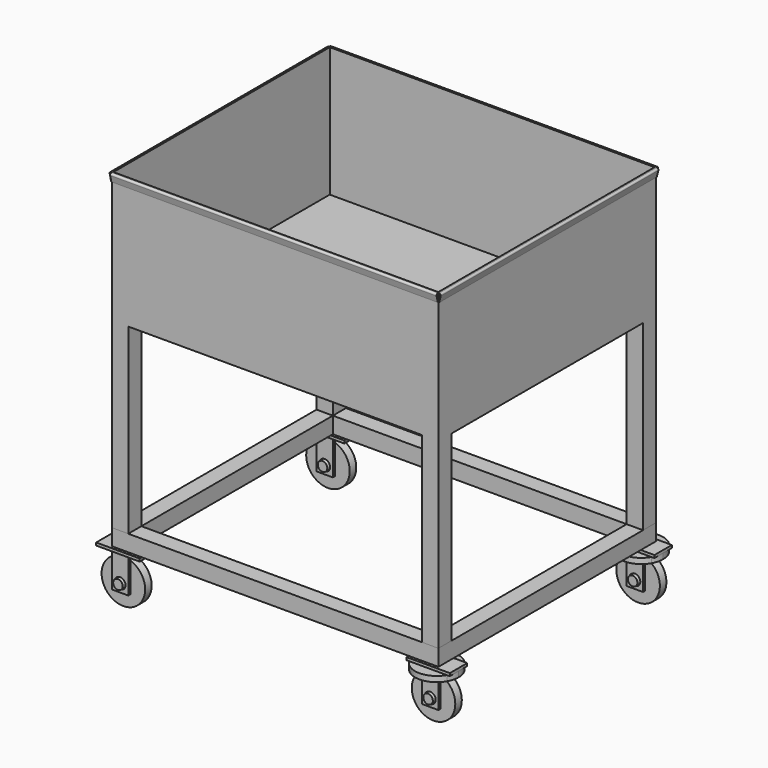
from build123d import *

# Parameters (mm, degrees)
F0_W             = 762
F0_H             = 635
F1_DEPTH         = 304.8
F2_T             = -1.89738
F3_W             = 38.1
F3_H             = 38.1
F3_W_2           = 25.4
F3_H_2           = 25.4
F4_DEPTH         = 463.8548
F5_W             = 101.6
F5_H             = 50.8
F5_W_2           = 38.1
F5_H_2           = 38.1
F5_W_3           = 25.4
F5_H_3           = 25.4
F6_DEPTH         = 6.35
F7_W             = 38.1
F7_H             = 88.9
F7_R             = 12.7
F8_DEPTH         = 6.35
F8_COPIES1_COUNT = 2
F8_COPIES1_PITCH = 724.595937
F11_R            = 50.8
F11_R_2          = 12.7
F12_DEPTH        = 9.525
F13_R            = 11.1125
F14_DEPTH        = 25.4
F18_DEPTH        = 12.7
F21_DEPTH        = 762
F23_DEPTH        = 635
F24_W            = 38.1
F24_H            = 38.1
F24_W_2          = 31.75
F24_H_2          = 6.35
F24_H_3          = 552.45
F25_DEPTH        = 38.1


# Not quite as in the source:
# - ends of sketch curves that miss each other by under 0.0002 mm in the source are joined
# - a pattern or mirror of a feature is missing from the dataset's text; its kind, count and spacing are read off the source's solid


with BuildPart() as f1:
    # F0 (on Top) → F1 (new body)
    with BuildSketch(Plane.XY):
        Rectangle(F0_W, F0_H)
    extrude(amount=F1_DEPTH)

    # F2
    f2_openings = [f1.faces().sort_by_distance(p)[0] for p in [
        (0, 0, 304.8),
    ]]
    offset(amount=F2_T, openings=f2_openings)

    # F4_copies: F4 across plane


with BuildPart() as f4:
    # F3 (on face) → F4 (new body)
    with BuildSketch(Plane(origin=(0, 0, 0), x_dir=(1, 0, 0), z_dir=(0, 0, -1))):
        with Locations((-361.95, 298.45)):
            Rectangle(F3_W, F3_H)
        with Locations((-361.95, 298.45)):
            Rectangle(F3_W_2, F3_H_2, mode=Mode.SUBTRACT)
    extrude(amount=F4_DEPTH)


with BuildPart() as f1_1:
    add(f1.part)
    add(f4.part.mirror(Plane(origin=(0, 0, 0), x_dir=(0, 0, 1), z_dir=(1, 0, 0))))

    # F6_copies: F6 across plane


with BuildPart() as f6:
    # F5 (on face) → F6 (new body)
    with BuildSketch(Plane(origin=(0, 0, -463.8548), x_dir=(1, 0, 0), z_dir=(0, 0, -1))):
        with Locations((-361.95, 298.45)):
            Rectangle(F5_W, F5_H)
        with Locations((-361.95, 298.45)):
            Rectangle(F5_W_2, F5_H_2, mode=Mode.SUBTRACT)
        with Locations((-361.95, 298.45)):
            Rectangle(F5_W_2, F5_H_2)
        with Locations((-361.95, 298.45)):
            Rectangle(F5_W_3, F5_H_3, mode=Mode.SUBTRACT)
        with Locations((-361.95, 298.45)):
            Rectangle(F5_W_3, F5_H_3)
    extrude(amount=F6_DEPTH)


with BuildPart() as f1_2:
    add(f1_1.part)
    add(f6.part.mirror(Plane(origin=(0, 0, 0), x_dir=(0, 0, 1), z_dir=(1, 0, 0))))

    # F8_copies: F8 across plane


with BuildPart() as f8:
    # F7 (on face) → F8 (new body)
    with BuildSketch(Plane.XZ.offset(317.5)):
        with Locations((-361.95, -508.3048)):
            Rectangle(F7_W, F7_H)
        with Locations((-361.95, -533.7048)):
            Circle(F7_R, mode=Mode.SUBTRACT)
    extrude(amount=-F8_DEPTH)


with BuildPart() as f1_3:
    add(f1_2.part)
    add(f8.part.mirror(Plane(origin=(0, 0, 0), x_dir=(0, 0, 1), z_dir=(1, 0, 0))))

    # F8_copies1: F8 ×2
    with Locations(*[Vector(0.9990395511, 0.0438175242, 0) * (i * F8_COPIES1_PITCH) for i in range(1, F8_COPIES1_COUNT)]):
        add(f8.part)

    # F15: F12, F8, F4, F14 across plane


with BuildPart() as f4_1:
    add(f4.part)

    add(f6.part)  # F10 merges F6
    # F10: F8 across plane
    add(f8.part.mirror(Plane(origin=(-361.95, -298.45, -467.0298), x_dir=(-1, 0, 0), z_dir=(0, 1, 0))))


with BuildPart() as f12:
    # F11 (on mid) → F12 (new body, symmetric)
    with BuildSketch(Plane(origin=(0, -298.45, 0), x_dir=(-1, 0, 0), z_dir=(0, 1, 0))):
        with Locations((361.95, -533.7048)):
            Circle(F11_R)
        with Locations((361.95, -533.7048)):
            Circle(F11_R_2, mode=Mode.SUBTRACT)
    extrude(amount=F12_DEPTH, both=True)


with BuildPart() as f14:
    # F13 (on mid) → F14 (new body, symmetric)
    with BuildSketch(Plane(origin=(0, -298.45, 0), x_dir=(-1, 0, 0), z_dir=(0, 1, 0))):
        with Locations((361.95, -533.7048)):
            Circle(F13_R)
    extrude(amount=F14_DEPTH, both=True)


with BuildPart() as f1_4:
    add(f1_3.part)
    add(f12.part.mirror(Plane.XZ))
    add(f8.part.mirror(Plane.XZ))
    add(f4_1.part.mirror(Plane.XZ))
    add(f14.part.mirror(Plane.XZ))



with BuildPart() as f1_5:
    add(f1_4.part)

    add(f4_1.part)  # F16 merges F4

    add(f8.part)  # F16 merges F8
    # F16: F12, F1, F14 across plane
    add(f12.part.mirror(Plane.YZ))
    add(f1_4.part.mirror(Plane.YZ))
    add(f14.part.mirror(Plane.YZ))


with BuildPart() as f18:
    # F17 (on face) → F18 (new body)
    with BuildSketch(Plane(origin=(0, 0, -470.2048), x_dir=(1, 0, 0), z_dir=(0, 0, -1))):
        with BuildLine():
            ThreePointArc((405.9440905122, -323.85), (411.0190319755, -311.5980074912), (412.75, -298.45))
            ThreePointArc((412.75, -298.45), (411.0190319755, -285.3019925088), (405.9440905122, -273.05))
            Line((405.9440905122, -273.05), (361.95, -273.05))
            Line((361.95, -273.05), (361.95, -279.4))
            Line((361.95, -279.4), (381, -279.4))
            Line((381, -279.4), (381, -285.75))
            Line((381, -285.75), (361.95, -285.75))
            Line((361.95, -285.75), (361.95, -311.15))
            Line((361.95, -311.15), (381, -311.15))
            Line((381, -311.15), (381, -317.5))
            Line((381, -317.5), (361.95, -317.5))
            Line((361.95, -317.5), (361.95, -323.85))
            Line((361.95, -323.85), (405.9440905122, -323.85))
        make_face()
        with BuildLine():
            Line((361.95, -273.05), (405.9440905122, -273.05))
            ThreePointArc((405.9440905122, -273.05), (361.95, -247.65), (317.9559094878, -273.05))
            Line((317.9559094878, -273.05), (361.95, -273.05))
        make_face()
        with BuildLine():
            ThreePointArc((317.9559094878, -323.85), (361.95, -349.25), (405.9440905122, -323.85))
            Line((405.9440905122, -323.85), (361.95, -323.85))
            Line((361.95, -323.85), (317.9559094878, -323.85))
        make_face()
        with BuildLine():
            Line((361.95, -273.05), (317.9559094878, -273.05))
            ThreePointArc((317.9559094878, -273.05), (312.8809680245, -285.3019925088), (311.15, -298.45))
            ThreePointArc((311.15, -298.45), (312.8809680245, -311.5980074912), (317.9559094878, -323.85))
            Line((317.9559094878, -323.85), (361.95, -323.85))
            Line((361.95, -323.85), (361.95, -317.5))
            Line((361.95, -317.5), (342.9, -317.5))
            Line((342.9, -317.5), (342.9, -311.15))
            Line((342.9, -311.15), (361.95, -311.15))
            Line((361.95, -311.15), (361.95, -285.75))
            Line((361.95, -285.75), (342.9, -285.75))
            Line((342.9, -285.75), (342.9, -279.4))
            Line((342.9, -279.4), (361.95, -279.4))
            Line((361.95, -279.4), (361.95, -273.05))
        make_face()
    extrude(amount=F18_DEPTH)


with BuildPart() as f19_1:
    # F19: instance of F18
    add(f18.part.mirror(Plane.XZ))


with BuildPart() as f21:
    # F20 (on face) → F21 (new body, through all)
    with BuildSketch(Plane(origin=(-381, 0, 0), x_dir=(0, -1, 0), z_dir=(-1, 0, 0))):
        with BuildLine():
            Line((-317.5, 302.90262), (-317.5, 304.8))
            Line((-317.5, 304.8), (-319.0535416211, 304.8))
            ThreePointArc((-319.0535416211, 304.8), (-322.0295428289, 303.359729386), (-322.7465094275, 300.1322037816))
            Line((-322.7465094275, 300.1322037816), (-319.3464839032, 285.75))
            Line((-319.3464839032, 285.75), (-317.5, 286.1865181092))
            Line((-317.5, 286.1865181092), (-320.9000255243, 300.5687218908))
            ThreePointArc((-320.9000255243, 300.5687218908), (-320.541542225, 302.182484693), (-319.0535416211, 302.90262))
            Line((-319.0535416211, 302.90262), (-317.5, 302.90262))
        make_face()
    extrude(amount=-F21_DEPTH)


with BuildPart() as f21b:
    # F20 (on face) → F21, piece 2 (new body, through all)
    with BuildSketch(Plane(origin=(-381, 0, 0), x_dir=(0, -1, 0), z_dir=(-1, 0, 0))):
        with BuildLine():
            Line((319.0535416211, 304.8), (317.5, 304.8))
            Line((317.5, 304.8), (317.5, 302.90262))
            Line((317.5, 302.90262), (319.0535416211, 302.90262))
            ThreePointArc((319.0535416211, 302.90262), (320.541542225, 302.182484693), (320.9000255243, 300.5687218908))
            Line((320.9000255243, 300.5687218908), (317.5, 286.1865181092))
            Line((317.5, 286.1865181092), (319.3464839032, 285.75))
            Line((319.3464839032, 285.75), (322.7465094275, 300.1322037816))
            ThreePointArc((322.7465094275, 300.1322037816), (322.0295428289, 303.359729386), (319.0535416211, 304.8))
        make_face()
    extrude(amount=-F21_DEPTH)


with BuildPart() as f23:
    # F22 (on face) → F23 (new body, through all)
    with BuildSketch(Plane(origin=(0, 317.5, 0), x_dir=(-1, 0, 0), z_dir=(0, 1, 0))):
        with BuildLine():
            Line((-381, 302.8843261488), (-381, 304.8))
            Line((-381, 304.8), (-383.1514110451, 304.5005266943))
            ThreePointArc((-383.1514110451, 304.5005266943), (-385.7621614566, 302.8817897377), (-386.3192742384, 299.860870607))
            Line((-386.3192742384, 299.860870607), (-382.8455219884, 285.3094328034))
            Line((-382.8455219884, 285.3094328034), (-381, 285.75))
            Line((-381, 285.75), (-384.47375225, 300.3014378036))
            ThreePointArc((-384.47375225, 300.3014378036), (-384.1951958591, 301.8118973689), (-382.8898206534, 302.6212658473))
            Line((-382.8898206534, 302.6212658473), (-381, 302.8843261488))
        make_face()
    extrude(amount=-F23_DEPTH)


with BuildPart() as f23b:
    # F22 (on face) → F23, piece 2 (new body, through all)
    with BuildSketch(Plane(origin=(0, 317.5, 0), x_dir=(-1, 0, 0), z_dir=(0, 1, 0))):
        with BuildLine():
            Line((383.1514110451, 304.5005266943), (381, 304.8))
            Line((381, 304.8), (381, 302.8843261488))
            Line((381, 302.8843261488), (382.8898206534, 302.6212658473))
            ThreePointArc((382.8898206534, 302.6212658473), (384.1951958591, 301.8118973689), (384.47375225, 300.3014378036))
            Line((384.47375225, 300.3014378036), (381, 285.75))
            Line((381, 285.75), (382.8455219884, 285.3094328034))
            Line((382.8455219884, 285.3094328034), (386.3192742384, 299.860870607))
            ThreePointArc((386.3192742384, 299.860870607), (385.7621614566, 302.8817897377), (383.1514110451, 304.5005266943))
        make_face()
    extrude(amount=-F23_DEPTH)


with BuildPart() as f25:
    # F24 (on face) → F25 (new body)
    with BuildSketch(Plane.XY.offset(-463.8548)):
        with Locations((-361.95, 298.45)):
            Rectangle(F24_W, F24_H)
        with Locations((-327.025, 298.45)):
            Rectangle(F24_W_2, F24_H)
        with Locations((-361.95, 276.225)):
            Rectangle(F24_W, F24_H_2)
        Polygon((381, 317.5), (-311.15, 317.5), (-311.15, 279.4), (342.9, 279.4), (342.9, -279.4), (-342.9, -279.4), (-342.9, -317.5), (381, -317.5), align=None)
        with Locations((-361.95, -3.175)):
            Rectangle(F24_W, F24_H_3)
        with Locations((-361.95, -298.45)):
            Rectangle(F24_W, F24_H)
    extrude(amount=F25_DEPTH)


solid = Compound([f12.part, f14.part, f1_5.part, f18.part, f19_1.part, f21.part, f21b.part, f23.part, f23b.part, f25.part])
